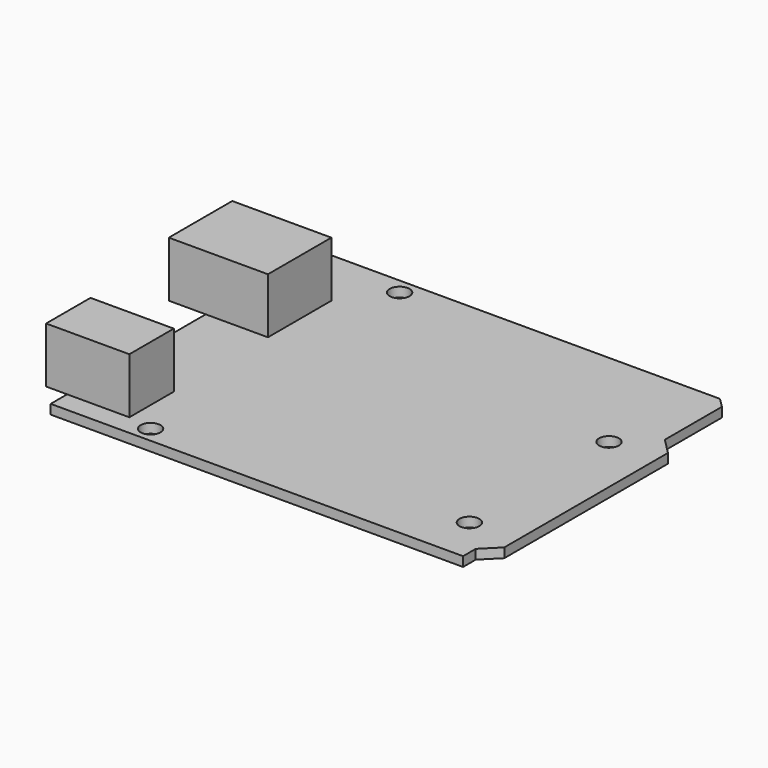
from build123d import *

# Parameters (mm, degrees)
F0_R     = 1.5875
F1_DEPTH = 1.524
F2_W     = 5.913735792
F2_H     = 12.7
F2_W_2   = 9.961264208
F2_W_3   = 3.373735792
F2_H_2   = 8.89
F3_DEPTH = 8.89


# Not quite as in the source:
# - a feature names something its author has since deleted; it is built from what else it names


with BuildPart() as f1:
    # F0 (on Top) → F1 (new body)
    with BuildSketch(Plane.XY):
        Polygon((0, 53.34), (0, 0), (66.04, 0), (66.04, 2.54), (68.58, 5.08), (68.58, 37.846), (66.04, 40.386), (66.04, 51.816), (64.516, 53.34), align=None)
        with Locations((13.97, 2.54)):
            Circle(F0_R, mode=Mode.SUBTRACT)
        with Locations((60.96, 7.62)):
            Circle(F0_R, mode=Mode.SUBTRACT)
        with Locations((15.24, 50.8)):
            Circle(F0_R, mode=Mode.SUBTRACT)
        with Locations((60.96, 35.56)):
            Circle(F0_R, mode=Mode.SUBTRACT)
    extrude(amount=-F1_DEPTH)

    # F2 (on face) → F3 (join)
    with BuildSketch(Plane.XY):
        with Locations((-2.956867896, 37.39)):
            Rectangle(F2_W, F2_H)
        with Locations((4.980632104, 37.39)):
            Rectangle(F2_W_2, F2_H)
        with Locations((-1.686867896, 7.745)):
            Rectangle(F2_W_3, F2_H_2)
        with Locations((4.980632104, 7.745)):
            Rectangle(F2_W_2, F2_H_2)
    extrude(amount=F3_DEPTH)


solid = f1.part
